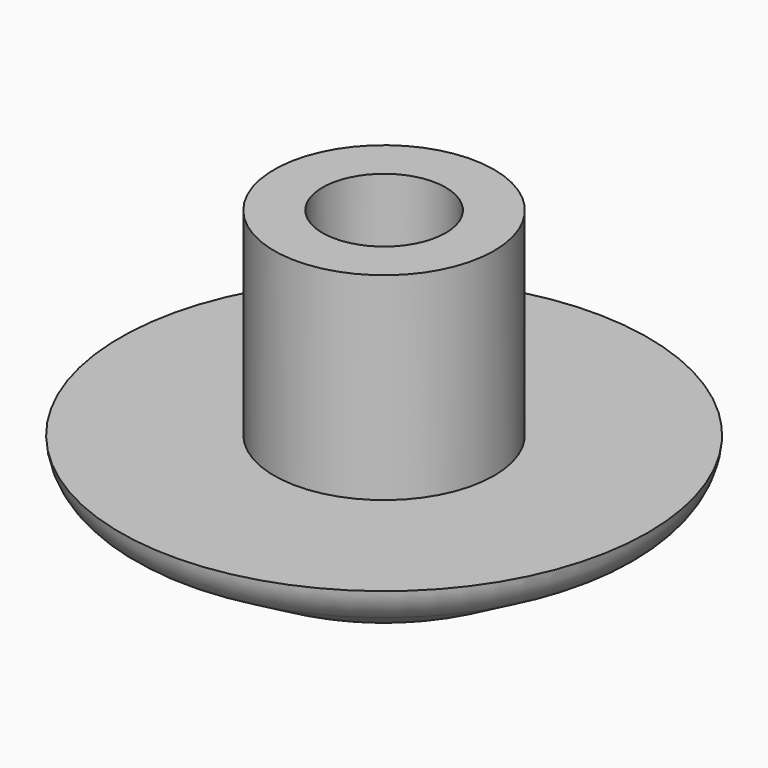
from build123d import *

# Parameters (mm, degrees)
F0_R     = 6
F1_DEPTH = 2
F2_SIZE2 = 2.5980762114
F2_SIZE  = 1.5
F4_R     = 2.5
F4_R_2   = 1.4
F5_DEPTH = 4.5
F6_R     = 1.2


# Not quite as in the source:
# - a fillet or chamfer that OpenCascade refuses, or shapes differently, is made with other operations: its cross-section is extruded or revolved along the edge and cut away or added


with BuildPart() as f1:
    # F0 (on Top) → F1 (new body)
    with BuildSketch(Plane.XY):
        Circle(F0_R)
    extrude(amount=F1_DEPTH)

    # F2
    f2_edges = [f1.edges().sort_by_distance(p)[0] for p in [
        (-6, 0, 0),
    ]]
    f2_side = f1.faces().sort_by_distance((-6, 0, 1))[0]
    chamfer(f2_edges, length=F2_SIZE, length2=F2_SIZE2, reference=f2_side)

    # F3: fillet of radius 1 on 2 edges, made by hand

    # F3_s1 → F3_t2 (revolve, cut)
    with BuildSketch(Plane.XZ):
        with BuildLine():
            ThreePointArc((3.6339745962, 0.1339745962), (3.3927936413, 0.0340741737), (3.1339745962, 0))
            Line((3.1339745962, 0), (3.4019237886, 0))
            Line((3.4019237886, 0), (3.6339745962, 0.1339745962))
        make_face()
    revolve(axis=Axis((0, 0, 0), (0, 0, 1)), mode=Mode.SUBTRACT)

    # F3_s3 → F3_t4 (revolve, cut)
    with BuildSketch(Plane.XZ):
        with BuildLine():
            ThreePointArc((6, 2), (5.8486778537, 1.5452494356), (5.5031382462, 1.2131367327))
            Line((5.5031382462, 1.2131367327), (6, 1.5))
            Line((6, 1.5), (6, 2))
        make_face()
    revolve(axis=Axis((0, 0, 1.5), (0, 0, 1)), mode=Mode.SUBTRACT)

    # F4 (on face) → F5 (join)
    with BuildSketch(Plane.XY.offset(2)):
        Circle(F4_R)
        Circle(F4_R_2, mode=Mode.SUBTRACT)
    extrude(amount=F5_DEPTH)

    # F6
    f6_edges = [f1.edges().sort_by_distance(p)[0] for p in [
        (-1.4, 0, 2),
    ]]
    fillet(f6_edges, radius=F6_R)


solid = f1.part
